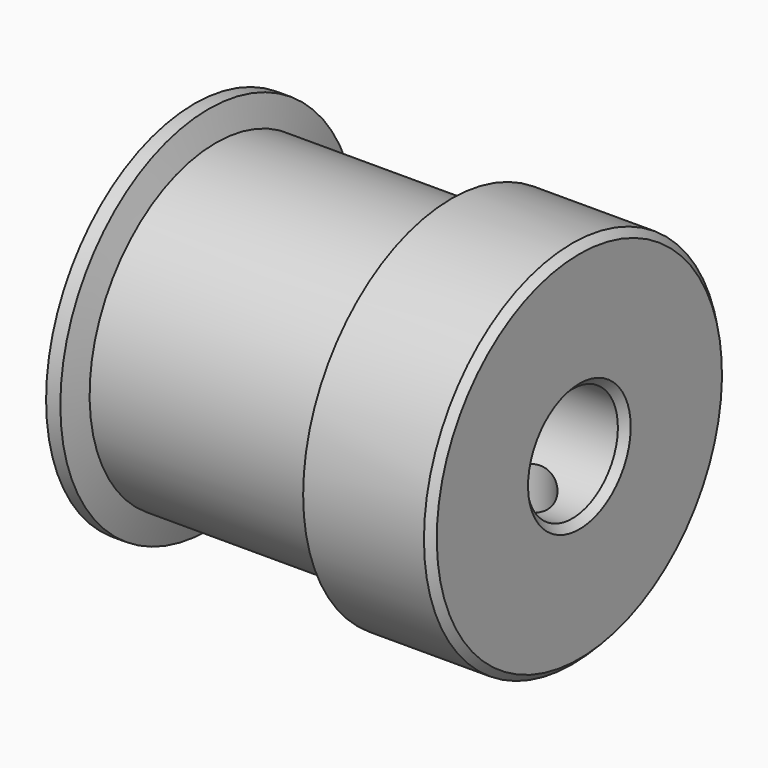
from build123d import *

# Parameters (mm, degrees)
F2_SIZE  = 0.5
F4_D     = 5
F4_DEPTH = 13.001


with BuildPart() as f1:
    # F0 (on Front) → F1 (revolve)
    with BuildSketch(Plane.XZ):
        Polygon((-8.9710751011, 13), (-9.4855375505, 11.08), (-25.4855375505, 11.08), (-26, 13), (-27, 13), (-26.4855375505, 11.08), (-26.4855375505, 8), (-27, 8), (-27, 4), (0, 4), (0, 13), align=None)
    revolve(axis=Axis((-13.5, 0, 0), (1, 0, 0)))

    # F2
    f2_edges = [f1.edges().sort_by_distance(p)[0] for p in [
        (0, 0, -4),
        (0, 0, -13),
        (-27, 0, -8),
        (-27, 0, -4),
    ]]
    chamfer(f2_edges, length=F2_SIZE)

    # F4 (through all, one way)
    with BuildSketch(Plane.XY):
        with Locations((-4.7355375505, 0)):
            Circle(F4_D / 2)
    extrude(amount=-F4_DEPTH, mode=Mode.SUBTRACT)


solid = f1.part
